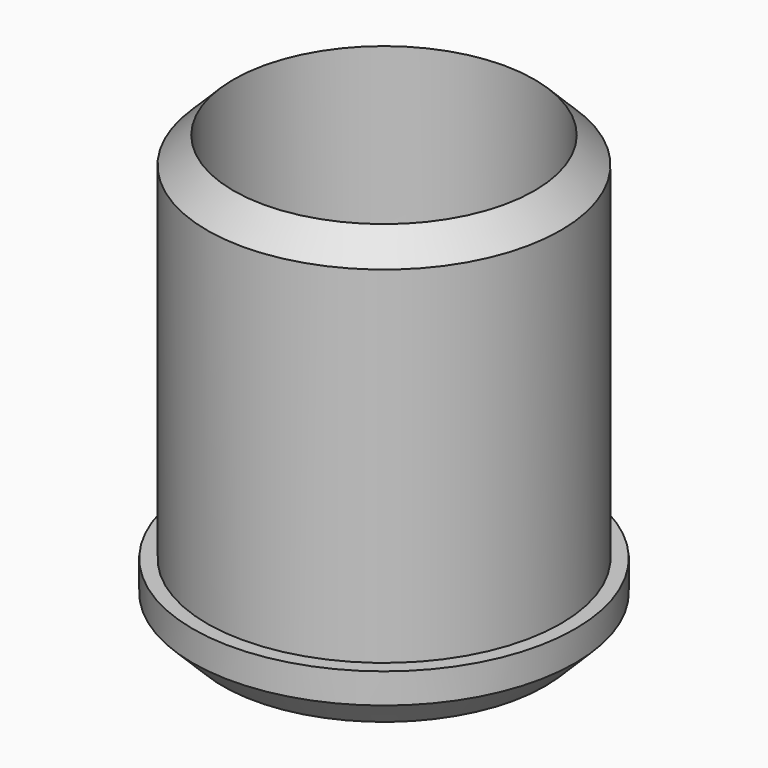
from build123d import *

# Parameters (mm, degrees)
F0_R     = 12.7
F0_R_2   = 11.75
F0_R_3   = 10
F1_DEPTH = 4
F2_DEPTH = 25


# Not quite as in the source:
# - a fillet or chamfer that OpenCascade refuses, or shapes differently, is made with other operations: its cross-section is extruded or revolved along the edge and cut away or added


with BuildPart() as f1:
    # F0 (on Top) → F1 (new body)
    with BuildSketch(Plane.XY):
        Circle(F0_R)
        Circle(F0_R_2, mode=Mode.SUBTRACT)
        Circle(F0_R_2)
        Circle(F0_R_3, mode=Mode.SUBTRACT)
        Circle(F0_R_3)
    extrude(amount=-F1_DEPTH)

    # F0 (on Top) → F2 (join)
    with BuildSketch(Plane.XY):
        Circle(F0_R_2)
        Circle(F0_R_3, mode=Mode.SUBTRACT)
    extrude(amount=F2_DEPTH)

    # F3: chamfer of 2 on 2 edges, made by hand

    # F3_s1 → F3_t2 (revolve, cut)
    with BuildSketch(Plane.XZ):
        Polygon((11.75, 23), (9.75, 25), (11.75, 25), align=None)
    revolve(axis=Axis((0, 0, 25), (0, 0, 1)), mode=Mode.SUBTRACT)

    # F3_s3 → F3_t4 (revolve, cut)
    with BuildSketch(Plane.XZ):
        Polygon((12.7, -2), (10.7, -4), (12.7, -4), align=None)
    revolve(axis=Axis((0, 0, -4), (0, 0, 1)), mode=Mode.SUBTRACT)


solid = f1.part
